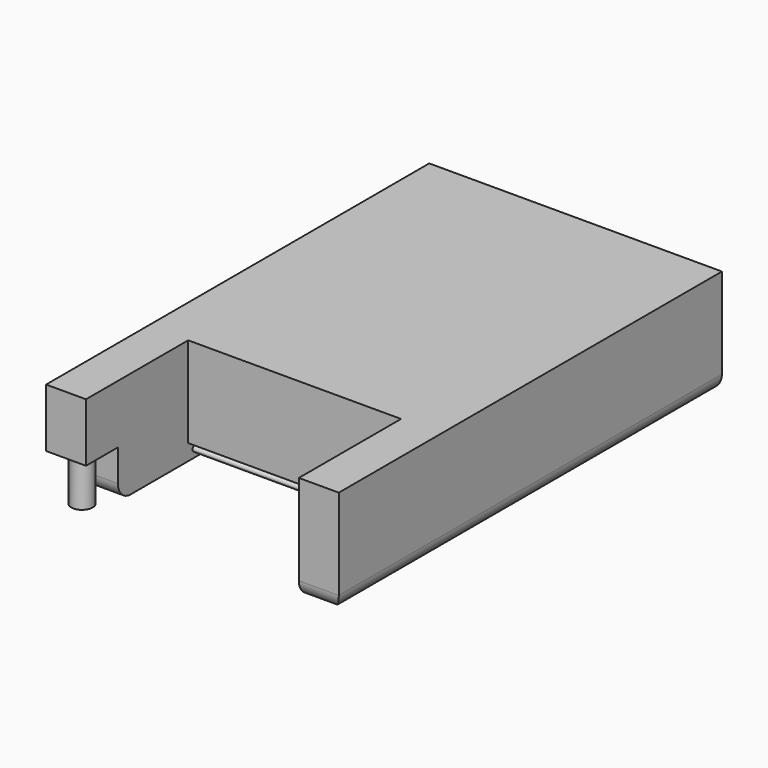
from build123d import *

# Parameters (mm, degrees)
F1_DEPTH = 100
F2_W     = 37.5
F2_H     = 37.5
F2_R     = 10
F3_DEPTH = 45
F4_W     = 200
F4_H     = 15
F5_DEPTH = 15
F6_R     = 2.5
F7_DEPTH = 200
F8_R     = 15


# Not quite as in the source:
# - a feature of the source that left no trace in its solid (it failed there, or was rolled back) is left out


with BuildPart() as f1:
    # F0 (on Top) → F1 (new body)
    with BuildSketch(Plane.XY):
        Polygon((137.5, 225), (-137.5, 225), (-137.5, -225), (-100, -225), (-100, -105), (100, -105), (100, -225), (137.5, -225), align=None)
    extrude(amount=F1_DEPTH)

    # F2 (on face) → F3 (cut)
    with BuildSketch(Plane(origin=(0, 0, 0), x_dir=(1, 0, 0), z_dir=(0, 0, -1))):
        with Locations((-118.75, 206.25)):
            Rectangle(F2_W, F2_H)
        with Locations((-118.75, 206.25)):
            Circle(F2_R, mode=Mode.SUBTRACT)
    extrude(amount=-F3_DEPTH, mode=Mode.SUBTRACT)

    # F4 (on face) → F5 (cut)
    with BuildSketch(Plane.XZ.offset(105)):
        with Locations((0, 7.5)):
            Rectangle(F4_W, F4_H)
    extrude(amount=-F5_DEPTH, mode=Mode.SUBTRACT)

    # F6 (on face) → F7 (join)
    with BuildSketch(Plane.YZ.offset(-100)):
        with Locations((-97.5, 7.5)):
            Circle(F6_R)
    extrude(amount=F7_DEPTH)

    # F8
    f8_edges = [f1.edges().sort_by_distance(p)[0] for p in [
        (118.75, -225, 0),
        (137.5, 0, 0),
        (-137.5, 18.75, 0),
        (-118.75, -187.5, 0),
    ]]
    fillet(f8_edges, radius=F8_R)


solid = f1.part
